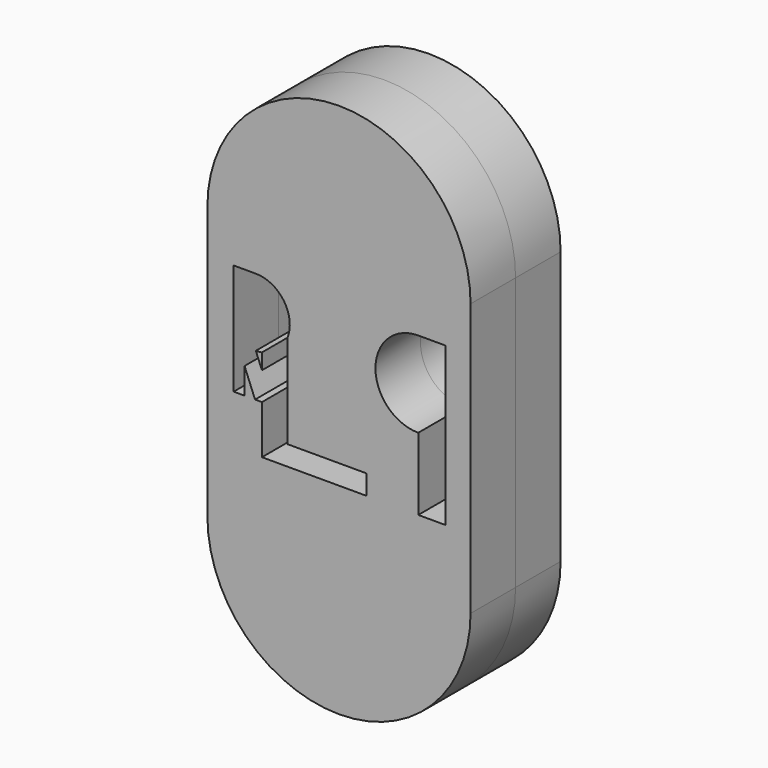
from build123d import *

# Parameters (mm, degrees)
F1_DEPTH = 25.4
F2_DEPTH = 25.4


with BuildPart() as f1:
    # F0 (on Front) → F1 (new body)
    with BuildSketch(Plane.XZ):
        with BuildLine():
            ThreePointArc((40.048032999, 69.6791410446), (-19.34594661, 129.0731206536), (-78.739926219, 69.6791410446))
            Line((-78.739926219, 69.6791410446), (-78.739926219, -53.3344708383))
            ThreePointArc((-78.739926219, -53.3344708383), (-19.34594661, -112.7284504473), (40.048032999, -53.3344708383))
            Line((40.048032999, -53.3344708383), (40.048032999, 69.6791410446))
        make_face()
        with BuildLine():
            Line((-54.1156261476, -21.8957141042), (-54.1156261476, 0))
            Line((-54.1156261476, 0), (-57.2257004678, 0))
            Line((-57.2257004678, 0), (-61.9756149655, 11.8043959837))
            Line((-61.9756149655, 11.8043959837), (-61.9756149655, 0))
            Line((-61.9756149655, 0), (-66.8679773808, 0))
            Line((-66.8679773808, 0), (-66.8679773808, 50.137385726))
            Line((-66.8679773808, 50.137385726), (-56.875812501, 50.137385726))
            ThreePointArc((-56.875812501, 50.137385726), (-44.1841953971, 43.3973306341), (-42.660497129, 29.1080398561))
            Line((-42.660497129, 29.1080398561), (-42.660497129, -12.968535535))
            Line((-42.660497129, -12.968535535), (-6.9517805241, -12.968535535))
            Line((-6.9517805241, -12.968535535), (-6.9517805241, -21.8957141042))
            Line((-6.9517805241, -21.8957141042), (-54.1156261476, -21.8957141042))
        make_face(mode=Mode.SUBTRACT)
        with BuildLine():
            ThreePointArc((16.4377391338, 10.7693783939), (-2.8852429241, 30.0923604518), (16.4377391338, 49.4153425097))
            Line((16.4377391338, 49.4153425097), (28.7177674472, 49.4153425097))
            Line((28.7177674472, 49.4153425097), (28.7177674472, -21.8957141042))
            Line((28.7177674472, -21.8957141042), (16.4377391338, -21.8957141042))
            Line((16.4377391338, -21.8957141042), (16.4377391338, 10.7693783939))
        make_face(mode=Mode.SUBTRACT)
    extrude(amount=F1_DEPTH)


with BuildPart() as f1b:
    # F0 (on Front) → F1, piece 2 (new body)
    with BuildSketch(Plane.XZ):
        with BuildLine():
            ThreePointArc((-54.1156261476, 19.7495529496), (-55.4900378278, 19.5616468515), (-56.875812501, 19.4988398184))
            Line((-56.875812501, 19.4988398184), (-54.1156261476, 12.6392778789))
            Line((-54.1156261476, 12.6392778789), (-54.1156261476, 19.7495529496))
        make_face()
    extrude(amount=F1_DEPTH)


with BuildPart() as f2:
    # F2 (new): a face of the model
    f2_faces = [f1.part.faces().sort_by_distance(p)[0] for p in [
        (-19.4720318388, -25.4, 7.0988838497),
    ]]
    extrude(f2_faces, amount=F2_DEPTH)


with BuildPart() as f2b:
    # F2#2 (new): a face of the model
    f2_2_faces = [f1b.part.faces().sort_by_distance(p)[0] for p in [
        (-55.0302076674, -25.4, 17.2683137212),
    ]]
    extrude(f2_2_faces, amount=F2_DEPTH)


solid = Compound([f1.part, f1b.part, f2.part, f2b.part])
